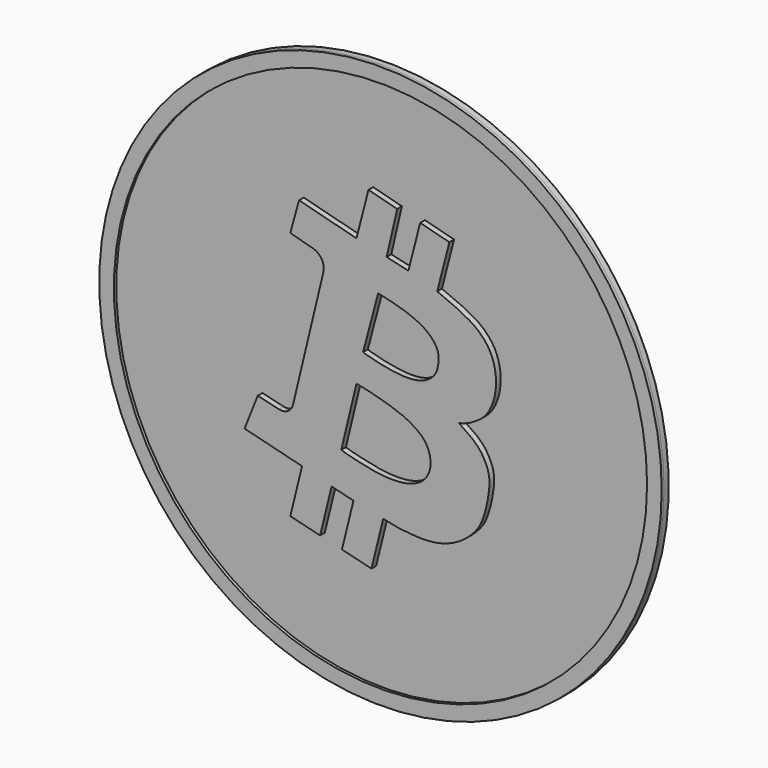
from build123d import *

# Parameters (mm, degrees)
F0_R     = 92
F1_DEPTH = 2
F3_DEPTH = 2
F4_SIZE  = 0.5
F5_R     = 96
F5_R_2   = 91
F6_DEPTH = 1
F7_R     = 96
F7_R_2   = 92.5
F8_DEPTH = 2


with BuildPart() as f1:
    # F0 (on Front) → F1 (new body)
    with BuildSketch(Plane.XZ):
        Circle(F0_R)
    extrude(amount=F1_DEPTH)

    # F2 (on face) → F3 (join)
    with BuildSketch(Plane.XZ.offset(2)):
        with BuildLine():
            Line((-27.0083267242, 47.4462620914), (-29.9760848284, 36.6564840078))
            Line((-29.9760848284, 36.6564840078), (-22.2285168536, 34.5254941518))
            ThreePointArc((-22.2285168536, 34.5254941518), (-19.2494475019, 32.2474077001), (-18.6923401828, 28.5387470903))
            Line((-18.6923401828, 28.5387470903), (-29.0434567348, -14.6331475965))
            ThreePointArc((-29.0434567348, -14.6331475965), (-30.842207656, -17.1104602787), (-33.8658412268, -17.5902759013))
            Line((-33.8658412268, -17.5902759013), (-41.0893774862, -15.8583235217))
            Line((-41.0893774862, -15.8583235217), (-45.5802306533, -27.2019170225))
            Line((-45.5802306533, -27.2019170225), (-25.9616385436, -32.1266614632))
            Line((-25.9616385436, -32.1266614632), (-29.9760848284, -48.441970569))
            Line((-29.9760848284, -48.441970569), (-19.817475765, -50.9415364766))
            Line((-19.817475765, -50.9415364766), (-15.8797713169, -34.9381176534))
            Line((-15.8797713169, -34.9381176534), (-8.4244611112, -36.7725261935))
            Line((-8.4244611112, -36.7725261935), (-12.3504317889, -52.7282572216))
            Line((-12.3504317889, -52.7282572216), (-2.2778489124, -55.2066560459))
            Line((-2.2778489124, -55.2066560459), (1.7324462003, -38.9082179233))
            add(Edge.make_bspline(
                [(27.6279114187, -1.7749243416), (28.7092025494, -2.4821118055), (30.7632053657, -3.8254734602), (33.1785734598, -5.7595776851), (35.5436051108, -8.3351168728), (37.6216996589, -12.4301034838), (38.2066856938, -16.2784704159), (37.5570764776, -21.1513349859), (36.6134428702, -25.4996695115), (35.0105992865, -30.2464913011), (32.2788072952, -33.64721937), (28.7034354961, -36.8048168389), (24.5561605745, -39.0157443509), (20.4502370232, -40.2644712402), (15.4624899933, -40.7624594383), (10.5521076326, -40.369441247), (6.0731193085, -39.9870515263), (3.1776998465, -39.2674221664), (1.7324462003, -38.9082179233)],
                knots=[0, 0, 0, 0, 0.0581811431, 0.1105199409, 0.166396485, 0.2299926025, 0.2891848852, 0.3549289053, 0.4189757736, 0.485313278, 0.5477155456, 0.6129869197, 0.6776623921, 0.7396069918, 0.8064894325, 0.8732457029, 0.9367303728, 1, 1, 1, 1], degree=3))
            add(Edge.make_bspline(
                [(20.1740991324, 35.3902466595), (21.6278121019, 34.6904285852), (24.3149738139, 33.6950984802), (29.3194313708, 31.4341194751), (34.3685495032, 28.396134608), (38.1341477981, 24.00928099), (39.9212139511, 19.2453405833), (40.5146903242, 13.7528029738), (39.3999313783, 7.8866877404), (36.7900227553, 3.1342771082), (33.4577982443, 0.7471944738), (30.842437236, -0.8483793153), (28.7242359185, -1.4589227998), (27.6279114187, -1.7749243416)],
                knots=[0, 0, 0, 0, 0.0879131849, 0.1842216609, 0.2852566372, 0.3837098851, 0.4762391657, 0.5729605468, 0.6742091416, 0.7698609916, 0.8525033329, 0.9244859802, 1, 1, 1, 1], degree=3))
            Line((20.1740991324, 35.3902466595), (24.3186354637, 51.5502765775))
            Line((24.3186354637, 51.5502765775), (14.3516925878, 54.1064820468))
            Line((14.3516925878, 54.1064820468), (10.3228697553, 38.3976325393))
            Line((10.3228697553, 38.3976325393), (2.8977939663, 40.1137321249))
            Line((2.8977939663, 40.1137321249), (6.511894986, 55.7509213686))
            Line((6.511894986, 55.7509213686), (-3.3063256055, 58.2813601075))
            Line((-3.3063256055, 58.2813601075), (-7.4012280942, 42.3929470361))
            Line((-7.4012280942, 42.3929470361), (-27.0083267242, 47.4462620914))
        make_face()
        with BuildLine():
            add(Edge.make_bspline(
                [(-7.3945214972, -1.2756045908), (-6.5768317056, -1.4028643234), (-4.63900586, -1.7427881734), (-2.57081296, -2.2995746446), (0.0421927128, -2.9636168954), (3.0184104723, -3.8011660264), (5.9488114617, -4.8226208543), (8.9704667551, -5.8952692635), (11.4440716652, -7.2485195874), (13.9774779434, -8.8724554322), (16.2131732777, -11.0678870183), (17.5644795402, -13.8713713722), (18.0569415504, -16.9841107708), (17.6084902929, -19.8814042944), (15.9556754656, -22.6059172587), (13.485660827, -24.5123892135), (9.5065873234, -25.9541132726), (4.911272628, -26.2048659523), (1.0813354306, -25.9598137418), (-2.7013841014, -25.417109761), (-5.5597148749, -24.7559847533), (-9.1231579206, -23.8913288849), (-10.6289368032, -23.5341618733), (-11.9050285979, -23.1026036338), (-12.5828394666, -22.8733764961)],
                knots=[0, 0, 0, 0, 0.0432107736, 0.0817951762, 0.1242054829, 0.1701874201, 0.2163611502, 0.2628601821, 0.3065968424, 0.3516498299, 0.3974950427, 0.44315253, 0.489019377, 0.5332628071, 0.5788489469, 0.6243879684, 0.6776568014, 0.7336079752, 0.7850652102, 0.8352687365, 0.881065134, 0.9301909347, 0.9629532558, 1, 1, 1, 1], degree=3))
            Line((-12.5828394666, -22.8733764961), (-7.3945214972, -1.2756045908))
        make_face(mode=Mode.SUBTRACT)
        with BuildLine():
            add(Edge.make_bspline(
                [(0, 28.2796639949), (0.6594507111, 28.1632733619), (2.0293480465, 27.8319072156), (4.4759400475, 27.312592786), (6.6129046687, 26.5807861519), (9.423953844, 25.9000782009), (12.1110497434, 24.7654919402), (14.8942249223, 23.6378539674), (18.1229068592, 21.1862173413), (20.5049371095, 18.1625957982), (20.7642688452, 14.5027255358), (20.0065708946, 10.3595714781), (17.154968946, 7.7981675266), (14.2040228218, 6.4857733605), (10.3534918094, 6.0512943472), (6.4301023642, 6.2721085581), (2.5706409463, 6.9434579896), (-0.9212078817, 7.6467920997), (-3.4708089675, 8.3887302885), (-4.6424710337, 8.6795403272), (-5.1260385662, 8.9294910431)],
                knots=[0, 0, 0, 0, 0.0451188564, 0.094356234, 0.1416763455, 0.194691, 0.2480920849, 0.3022750925, 0.3651943655, 0.4256230889, 0.4846354637, 0.547888998, 0.6075615518, 0.6634490372, 0.7245455133, 0.7868925643, 0.8491009373, 0.9085462245, 0.9592924665, 1, 1, 1, 1], degree=3))
            Line((-5.1260385662, 8.9294910431), (0, 28.2796639949))
        make_face(mode=Mode.SUBTRACT)
    extrude(amount=F3_DEPTH)

    # F4
    f4_edges = [f1.edges().sort_by_distance(p)[0] for p in [
        (-92, -2, 0),
    ]]
    chamfer(f4_edges, length=F4_SIZE)


with BuildPart() as f6:
    # F5 (on face) → F6 (new body)
    with BuildSketch(Plane.XZ.offset(2)):
        Circle(F5_R)
        Circle(F5_R_2, mode=Mode.SUBTRACT)
    extrude(amount=F6_DEPTH)

    # F7 (on face) → F8 (join)
    with BuildSketch(Plane(origin=(0, -2, 0), x_dir=(-1, 0, 0), z_dir=(0, 1, 0))):
        Circle(F7_R)
        Circle(F7_R_2, mode=Mode.SUBTRACT)
    extrude(amount=F8_DEPTH)


solid = Compound([f1.part, f6.part])
